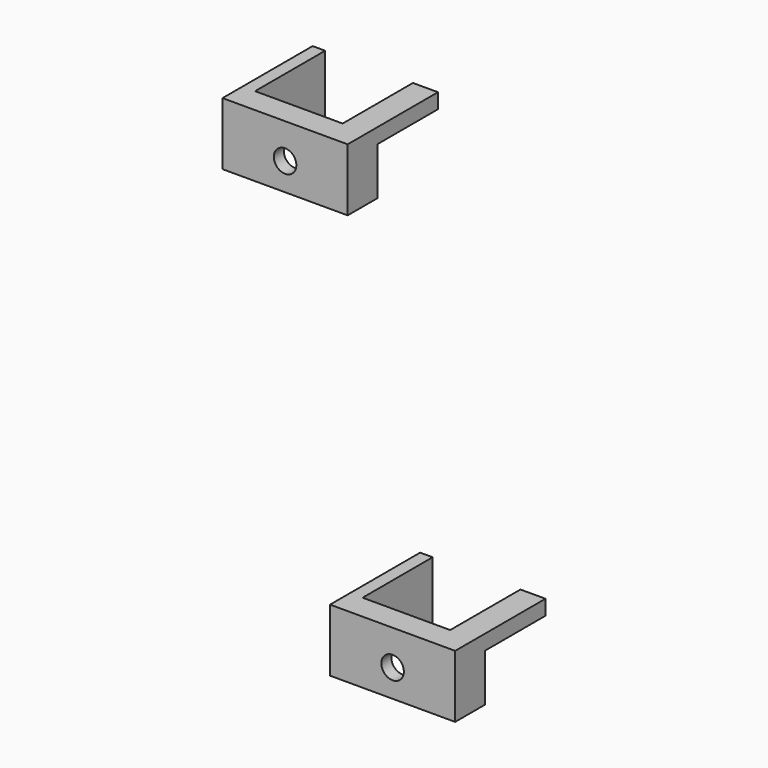
from build123d import *

# Parameters (mm, degrees)
F0_W      = 5
F0_H      = 30
F1_DEPTH  = 25
F2_W      = 5
F2_H      = 10
F3_DEPTH  = 5
F4_W      = 40
F4_H      = 25
F4_W_2    = 24
F4_H_2    = 15
F5_DEPTH  = 2
F7_DEPTH  = 49
F8_W      = 5
F8_H      = 1
F9_DEPTH  = 45.1
F4_R      = 4.5
F10_DEPTH = 25


# Not quite as in the source:
# - a feature names something its author has since deleted; it is built from what else it names


with BuildPart() as f1:
    # F0 (on Top) → F1 (new body)
    with BuildSketch(Plane.XY):
        Polygon((0, 15), (0, 0), (50, 0), (50, 15), (45, 15), (45, 5), (5, 5), (5, 15), align=None)
        with Locations((2.5, 30)):
            Rectangle(F0_W, F0_H)
    extrude(amount=F1_DEPTH)

    # F2 (on face) → F3 (join)
    with BuildSketch(Plane.XY.offset(25)):
        with Locations((47.5, 20)):
            Rectangle(F2_W, F2_H)
    extrude(amount=-F3_DEPTH)

    # F4 (on face) → F5 (join)
    with BuildSketch(Plane(origin=(0, 5, 0), x_dir=(-1, 0, 0), z_dir=(0, 1, 0))):
        with Locations((-25, 12.5)):
            Rectangle(F4_W, F4_H)
        with Locations((-25, 12.5)):
            Rectangle(F4_W_2, F4_H_2, mode=Mode.SUBTRACT)
    extrude(amount=F5_DEPTH)

    # F6 (on face) → F7 (join)
    with BuildSketch(Plane(origin=(0, 0, 0), x_dir=(0, -1, 0), z_dir=(-1, 0, 0))):
        with BuildLine():
            Line((-5, 19), (-5, 25))
            Line((-5, 25), (-10, 25))
            Line((-10, 25), (-10, 24))
            ThreePointArc((-10, 24), (-6.4644660941, 22.5355339059), (-5, 19))
        make_face()
    extrude(amount=-F7_DEPTH)

    # F8 (on face) → F9 (join)
    with BuildSketch(Plane.XZ):
        with BuildLine():
            Line((45, 19), (45, 24))
            Line((45, 24), (40, 24))
            ThreePointArc((40, 24), (41.4644660941, 20.4644660941), (45, 19))
        make_face()
        with Locations((42.5, 24.5)):
            Rectangle(F8_W, F8_H)
        Polygon((50, 19), (50, 25), (45, 25), (45, 24), (45, 19), align=None)
    extrude(amount=-F9_DEPTH)

    # F4 (on face) → F10 (cut)
    with BuildSketch(Plane(origin=(0, 5, 0), x_dir=(-1, 0, 0), z_dir=(0, 1, 0))):
        with Locations((-25, 11)):
            Circle(F4_R)
    extrude(amount=-F10_DEPTH, mode=Mode.SUBTRACT)


with BuildPart() as f11_1:
    # F11: copy of F1
    add(f1.part.moved(Location((0, -53.7, 200))))


solid = Compound([f1.part, f11_1.part])
